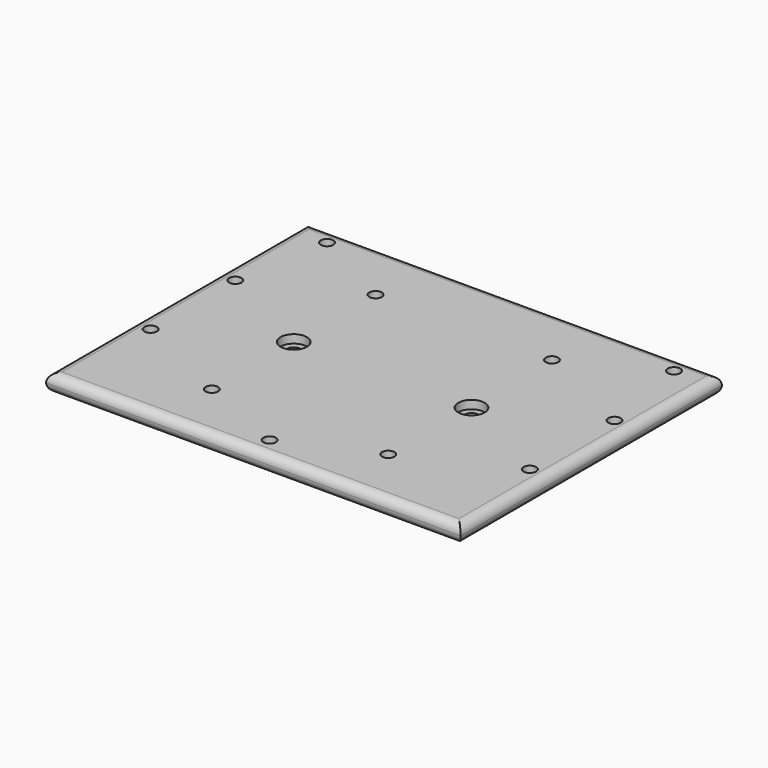
from build123d import *

# Parameters (mm, degrees)
F0_W      = 152.4
F0_H      = 127
F1_DEPTH  = 6.35
F2_R      = 2.25
F3_DEPTH  = 6.351
F4_R      = 2.5
F5_DEPTH  = 25.4
F6_R      = 4.75
F7_DEPTH  = 3
F8_R      = 2.2479
F9_DEPTH  = 6.351
F10_W     = 3.175
F10_H     = 9.42
F10_W_2   = 149.225
F10_H_2   = 117.58
F11_DEPTH = 6.351
F12_R     = 3.17499
F13_R     = 3.571875
F14_DEPTH = 2.54


# Not quite as in the source:
# - a fillet or chamfer is up to 0.001 mm smaller than in the source, because OpenCascade refuses the exact size


with BuildPart() as f1:
    # F0 (on Top) → F1 (new body)
    with BuildSketch(Plane.XY):
        with Locations((76.2, 63.5)):
            Rectangle(F0_W, F0_H)
    extrude(amount=F1_DEPTH)

    # F2 (on face) → F3 (cut, through all)
    with BuildSketch(Plane.XY.offset(6.35)):
        with Locations((15.3375, 120.65)):
            Circle(F2_R)
        with Locations((140.2375, 120.65)):
            Circle(F2_R)
        with Locations((77.7875, 16.75)):
            Circle(F2_R)
    extrude(amount=-F3_DEPTH, mode=Mode.SUBTRACT)

    # F4 (on face) → F5 (cut)
    with BuildSketch(Plane(origin=(0, 0, 0), x_dir=(1, 0, 0), z_dir=(0, 0, -1))):
        with Locations((45.7875, -67.575)):
            Circle(F4_R)
        with Locations((109.7875, -67.575)):
            Circle(F4_R)
    extrude(amount=-F5_DEPTH, mode=Mode.SUBTRACT)

    # F6 (on face) → F7 (cut)
    with BuildSketch(Plane.XY.offset(6.35)):
        with Locations((45.7875, 67.575)):
            Circle(F6_R)
        with Locations((109.7875, 67.575)):
            Circle(F6_R)
    extrude(amount=-F7_DEPTH, mode=Mode.SUBTRACT)

    # F8 (on face) → F9 (cut, through all)
    with BuildSketch(Plane.XY.offset(6.35)):
        with Locations((146.05, 86.625)):
            Circle(F8_R)
        with Locations((146.05, 48.525)):
            Circle(F8_R)
        with Locations((9.525, 48.525)):
            Circle(F8_R)
        with Locations((9.525, 86.625)):
            Circle(F8_R)
        with Locations((45.7875, 104.405)):
            Circle(F8_R)
        with Locations((109.2875, 104.405)):
            Circle(F8_R)
        with Locations((45.7875, 30.745)):
            Circle(F8_R)
        with Locations((109.2875, 30.745)):
            Circle(F8_R)
    extrude(amount=-F9_DEPTH, mode=Mode.SUBTRACT)

    # F10 (on face) → F11 (cut, through all)
    with BuildSketch(Plane.XY.offset(6.35)):
        with Locations((1.5875, 4.71)):
            Rectangle(F10_W, F10_H)
        with Locations((77.7875, 4.71)):
            Rectangle(F10_W_2, F10_H)
        with Locations((1.5875, 68.21)):
            Rectangle(F10_W, F10_H_2)
    extrude(amount=-F11_DEPTH, mode=Mode.SUBTRACT)

    # F12 (radius 3.175 in the source; OpenCascade refuses exactly that, so slightly less here)
    f12_edges = [f1.edges().sort_by_distance(p)[0] for p in [
        (3.175, 68.21, 6.35),
        (77.7875, 9.42, 6.35),
        (152.4, 68.21, 6.35),
        (77.7875, 127, 6.35),
        (77.7875, 127, 0),
        (3.175, 68.21, 0),
        (77.7875, 9.42, 0),
        (152.4, 68.21, 0),
    ]]
    fillet(f12_edges, radius=F12_R)

    # F13 (on face) → F14 (cut)
    with BuildSketch(Plane.XY):
        with Locations((45.7875, 30.745)):
            Circle(F13_R)
        with Locations((109.2875, 30.745)):
            Circle(F13_R)
        with Locations((9.525, 48.525)):
            Circle(F13_R)
        with Locations((9.525, 86.625)):
            Circle(F13_R)
        with Locations((45.7875, 104.405)):
            Circle(F13_R)
        with Locations((109.2875, 104.405)):
            Circle(F13_R)
        with Locations((146.05, 86.625)):
            Circle(F13_R)
        with Locations((146.05, 48.525)):
            Circle(F13_R)
    extrude(amount=F14_DEPTH, mode=Mode.SUBTRACT)


solid = f1.part
